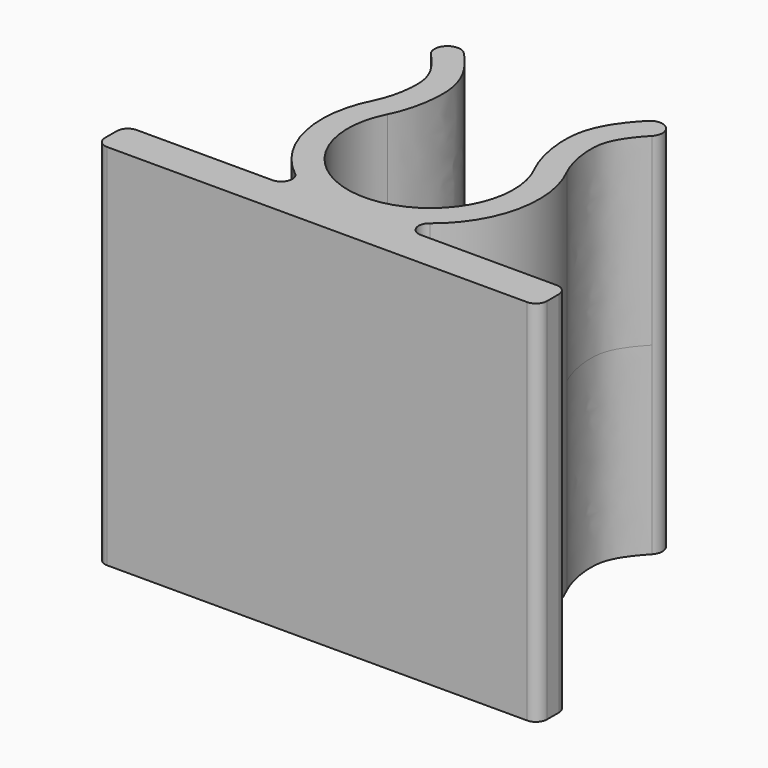
from build123d import *

# Parameters (mm, degrees)
F1_DEPTH = 5
F2_R     = 0.3


with BuildPart() as f1:
    # F0 (on Top) → F1 (new body, symmetric)
    with BuildSketch(Plane.XY):
        with BuildLine():
            ThreePointArc((2, 1.0307764064), (0, -2.25), (-2, 1.0307764064))
            add(Edge.make_bspline(
                [(-2, 1.0307764064), (-1.7928318797, 1.4327416027), (-1.4752005994, 2.7539357485), (-1.94238935, 3.6588384503), (-2.4898940219, 4.2405549061)],
                knots=[0, 0, 0, 0, 0.4856533037, 1, 1, 1, 1], degree=3))
            ThreePointArc((-2.4898940219, 4.2405549061), (-2.9846417573, 4.255544178), (-2.9996310293, 3.7607964426))
            add(Edge.make_bspline(
                [(-2.6222222222, 1.3514623995), (-2.5879840781, 1.4178941569), (-2.5120919735, 1.5965615902), (-2.4185643331, 1.9365442889), (-2.3646202091, 2.2979855215), (-2.3625995138, 2.6240888033), (-2.4081716924, 2.8742683693), (-2.5044815542, 3.1179920879), (-2.6847308977, 3.4036360851), (-2.8805852991, 3.6343119324), (-2.9996310293, 3.7607964426)],
                knots=[0, 0, 0, 0, 0.125, 0.25, 0.375, 0.5, 0.625, 0.75, 0.875, 1, 1, 1, 1], degree=3))
            ThreePointArc((-2.6222222222, 1.3514623995), (-2.6973313466, -1.1945307057), (-0.7615773106, -2.85))
            Line((-0.7615773106, -2.85), (0.7615773106, -2.85))
            ThreePointArc((0.7615773106, -2.85), (2.6973313466, -1.1945307057), (2.6222222222, 1.3514623995))
            add(Edge.make_bspline(
                [(2.6222222222, 1.3514623995), (2.5879840781, 1.4178941569), (2.5120919735, 1.5965615902), (2.4185643331, 1.9365442889), (2.3646202091, 2.2979855215), (2.3625995138, 2.6240888033), (2.4081716924, 2.8742683693), (2.5044815542, 3.1179920879), (2.6847308977, 3.4036360851), (2.8805852991, 3.6343119324), (2.9996310293, 3.7607964426)],
                knots=[0, 0, 0, 0, 0.125, 0.25, 0.375, 0.5, 0.625, 0.75, 0.875, 1, 1, 1, 1], degree=3))
            ThreePointArc((2.9996310293, 3.7607964426), (2.9846417573, 4.255544178), (2.4898940219, 4.2405549061))
            add(Edge.make_bspline(
                [(2, 1.0307764064), (1.7928318797, 1.4327416027), (1.4752005994, 2.7539357485), (1.94238935, 3.6588384503), (2.4898940219, 4.2405549061)],
                knots=[0, 0, 0, 0, 0.4856533037, 1, 1, 1, 1], degree=3))
        make_face()
        with BuildLine():
            ThreePointArc((0.7615773106, -2.85), (0, -2.95), (-0.7615773106, -2.85))
            Line((-0.7615773106, -2.85), (-6, -2.85))
            Line((-6, -2.85), (-6, -3.85))
            Line((-6, -3.85), (6, -3.85))
            Line((6, -3.85), (6, -2.85))
            Line((6, -2.85), (0.7615773106, -2.85))
        make_face()
        with BuildLine():
            Line((0.7615773106, -2.85), (-0.7615773106, -2.85))
            ThreePointArc((-0.7615773106, -2.85), (0, -2.95), (0.7615773106, -2.85))
        make_face()
    extrude(amount=F1_DEPTH, both=True)

    # F2
    f2_edges = [f1.edges().sort_by_distance(p)[0] for p in [
        (-6, -2.85, 0),
        (-6, -3.85, 0),
        (6, -2.85, 0),
        (6, -3.85, 0),
        (0.761577, -2.85, 0),
        (-0.761577, -2.85, 0),
    ]]
    fillet(f2_edges, radius=F2_R)


solid = f1.part
